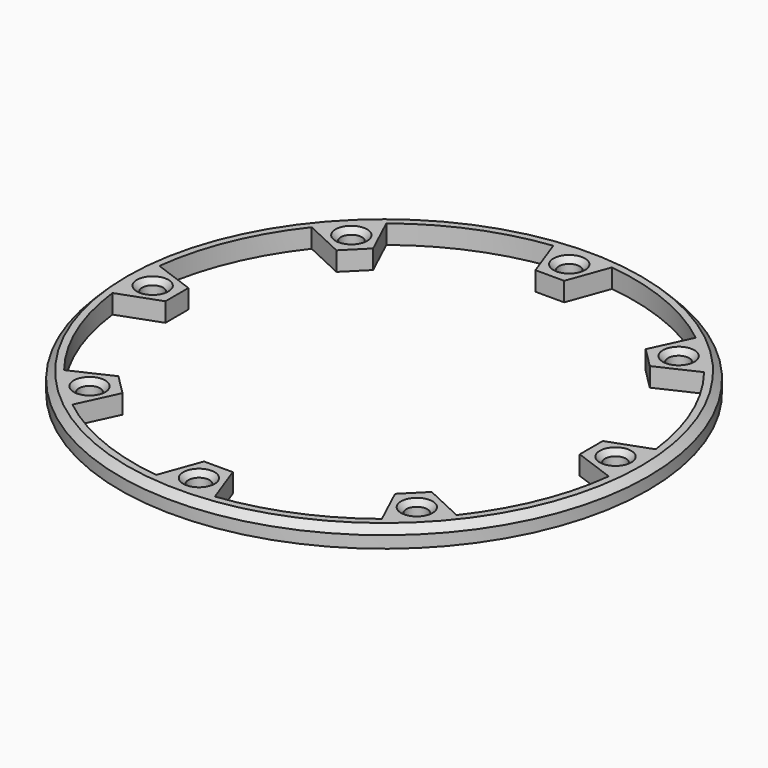
from build123d import *

# Parameters (mm, degrees)
F0_R            = 75
F1_DEPTH        = 5.4
F3_D            = 6
F3_DEPTH        = 6
F3_CSINK_D      = 8.96
F3_CSINK_ANGLE  = 90
F3_TIP          = 1.8025818571
F3_COPIES_COUNT = 8
F4_SIZE         = 2


# Not quite as in the source:
# - a pattern or mirror of a feature is missing from the dataset's text; its kind, count and spacing are read off the source's solid


with BuildPart() as f1:
    # F0 (on Top) → F1 (new body)
    with BuildSketch(Plane.XY):
        Circle(F0_R)
        with BuildLine():
            ThreePointArc((-70.5093388309, 8.3326654013), (-65.5954479473, 27.1705241697), (-55.749715835, 43.9655474137))
            Line((-55.749715835, 43.9655474137), (-44.5127719526, 38.7256744271))
            Line((-44.5127719526, 38.7256744271), (-38.7256744271, 44.5127719526))
            Line((-38.7256744271, 44.5127719526), (-43.9655474137, 55.749715835))
            ThreePointArc((-43.9655474137, 55.749715835), (-27.1705241697, 65.5954479473), (-8.3326654013, 70.5093388309))
            Line((-8.3326654013, 70.5093388309), (-4.0920959037, 58.8584698905))
            Line((-4.0920959037, 58.8584698905), (4.0920959037, 58.8584698905))
            Line((4.0920959037, 58.8584698905), (8.3326654013, 70.5093388309))
            ThreePointArc((8.3326654013, 70.5093388309), (27.1705241697, 65.5954479473), (43.9655474137, 55.749715835))
            Line((43.9655474137, 55.749715835), (38.7256744271, 44.5127719526))
            Line((38.7256744271, 44.5127719526), (44.5127719526, 38.7256744271))
            Line((44.5127719526, 38.7256744271), (55.749715835, 43.9655474137))
            ThreePointArc((55.749715835, 43.9655474137), (65.5954479473, 27.1705241697), (70.5093388309, 8.3326654013))
            Line((70.5093388309, 8.3326654013), (58.8584698905, 4.0920959037))
            Line((58.8584698905, 4.0920959037), (58.8584698905, -4.0920959037))
            Line((58.8584698905, -4.0920959037), (70.5093388309, -8.3326654013))
            ThreePointArc((70.5093388309, -8.3326654013), (65.5954479473, -27.1705241697), (55.749715835, -43.9655474137))
            Line((55.749715835, -43.9655474137), (44.5127719526, -38.7256744271))
            Line((44.5127719526, -38.7256744271), (38.7256744271, -44.5127719526))
            Line((38.7256744271, -44.5127719526), (43.9655474137, -55.749715835))
            ThreePointArc((43.9655474137, -55.749715835), (27.1705241697, -65.5954479473), (8.3326654013, -70.5093388309))
            Line((8.3326654013, -70.5093388309), (4.0920959037, -58.8584698905))
            Line((4.0920959037, -58.8584698905), (-4.0920959037, -58.8584698905))
            Line((-4.0920959037, -58.8584698905), (-8.3326654013, -70.5093388309))
            ThreePointArc((-8.3326654013, -70.5093388309), (-27.1705241697, -65.5954479473), (-43.9655474137, -55.749715835))
            Line((-43.9655474137, -55.749715835), (-38.7256744271, -44.5127719526))
            Line((-38.7256744271, -44.5127719526), (-44.5127719526, -38.7256744271))
            Line((-44.5127719526, -38.7256744271), (-55.749715835, -43.9655474137))
            ThreePointArc((-55.749715835, -43.9655474137), (-65.5954479473, -27.1705241697), (-70.5093388309, -8.3326654013))
            Line((-70.5093388309, -8.3326654013), (-58.8584698905, -4.0920959037))
            Line((-58.8584698905, -4.0920959037), (-58.8584698905, 4.0920959037))
            Line((-58.8584698905, 4.0920959037), (-70.5093388309, 8.3326654013))
        make_face(mode=Mode.SUBTRACT)
    extrude(amount=F1_DEPTH)

    # F3
    with Locations(Plane.XY.offset(5.4)):
        with Locations((-65.758, 0)):
            f3 = CounterSinkHole(F3_D / 2, F3_CSINK_D / 2, depth=F3_DEPTH, counter_sink_angle=F3_CSINK_ANGLE)
            with Locations((0, 0, -(F3_DEPTH + F3_TIP / 2))):  # 118° drill point
                Cone(0, F3_D / 2, F3_TIP, mode=Mode.SUBTRACT)

    # F3_copies: F3 ×8 about axis
    f3_copies_axis = Axis((0, 0, 0), (0, 0, 1))
    for i in range(1, F3_COPIES_COUNT):
        add(f3.rotate(f3_copies_axis, i * 360 / F3_COPIES_COUNT), mode=Mode.SUBTRACT)

    # F4
    f4_edges = [f1.edges().sort_by_distance(p)[0] for p in [
        (-75, 0, 5.4),
    ]]
    chamfer(f4_edges, length=F4_SIZE)


solid = f1.part
